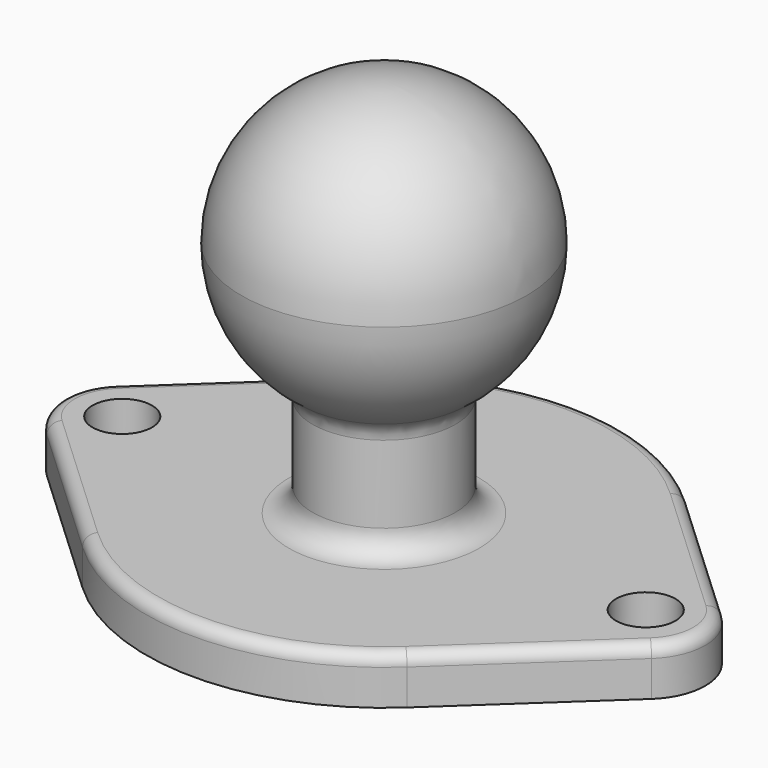
from build123d import *

# Parameters (mm, degrees)
F0_R     = 3.96875
F1_DEPTH = 6.35
F4_DEPTH = 15.2522160579
F5_R     = 1.6002
F6_R     = 3.175


with BuildPart() as f1:
    # F0 (on Top) → F1 (new body)
    with BuildSketch(Plane.XY):
        with BuildLine():
            Line((40.3369318182, 5.8064533276), (21.6477272727, 23.2258133103))
            ThreePointArc((21.6477272727, 23.2258133103), (11.6327754082, 29.5421907837), (0, 31.75))
            ThreePointArc((0, 31.75), (-11.6327754082, 29.5421907837), (-21.6477272727, 23.2258133103))
            Line((-21.6477272727, 23.2258133103), (-40.3369318182, 5.8064533276))
            ThreePointArc((-40.3369318182, 5.8064533276), (-42.8625, 0), (-40.3369318182, -5.8064533276))
            Line((-40.3369318182, -5.8064533276), (-21.6477272727, -23.2258133103))
            ThreePointArc((-21.6477272727, -23.2258133103), (0, -31.75), (21.6477272727, -23.2258133103))
            Line((21.6477272727, -23.2258133103), (40.3369318182, -5.8064533276))
            ThreePointArc((40.3369318182, -5.8064533276), (42.8625, 0), (40.3369318182, 5.8064533276))
        make_face()
        with Locations((-34.925, 0)):
            Circle(F0_R, mode=Mode.SUBTRACT)
        with BuildLine():
            ThreePointArc((9.525, 0), (-6.7351920908, -6.7351920908), (0, 9.525))
            ThreePointArc((0, 9.525), (6.7351920908, 6.7351920908), (9.525, 0))
        make_face(mode=Mode.SUBTRACT)
        with BuildLine():
            ThreePointArc((38.89375, 0), (34.925, -3.96875), (30.95625, 0))
            ThreePointArc((30.95625, 0), (34.925, 3.96875), (38.89375, 0))
        make_face(mode=Mode.SUBTRACT)
        with BuildLine():
            Line((0, 0), (0, 9.525))
            ThreePointArc((0, 9.525), (-6.7351920908, -6.7351920908), (9.525, 0))
            Line((9.525, 0), (0, 0))
        make_face()
        with BuildLine():
            ThreePointArc((9.525, 0), (6.7351920908, 6.7351920908), (0, 9.525))
            Line((0, 9.525), (0, 0))
            Line((0, 0), (9.525, 0))
        make_face()
    extrude(amount=-F1_DEPTH)



with BuildPart() as f3:
    # F2 (on Front) → F3 (revolve)
    with BuildSketch(Plane.XZ):
        with BuildLine():
            Line((0, 50.8), (0, 12.7))
            ThreePointArc((0, 12.7), (13.4703841816, 18.2796158184), (19.05, 31.75))
            ThreePointArc((19.05, 31.75), (13.4703841816, 45.2203841816), (0, 50.8))
        make_face()
    revolve(axis=Axis((0, 0, 25.4), (0, 0, 1)))


with BuildPart() as f1_1:
    add(f1.part)

    add(f3.part)  # F4 merges F3
    # F0 (on Top) → F4 (join, through all)
    with BuildSketch(Plane.XY):
        with BuildLine():
            Line((0, 0), (0, 9.525))
            ThreePointArc((0, 9.525), (-6.7351920908, -6.7351920908), (9.525, 0))
            Line((9.525, 0), (0, 0))
        make_face()
        with BuildLine():
            ThreePointArc((9.525, 0), (6.7351920908, 6.7351920908), (0, 9.525))
            Line((0, 9.525), (0, 0))
            Line((0, 0), (9.525, 0))
        make_face()
    extrude(amount=F4_DEPTH)

    # F5
    f5_edges = [f1_1.edges().sort_by_distance(p)[0] for p in [
        (0, -31.75, 0),
        (42.8625, 0, 0),
        (30.99233, -14.516133, 0),
        (30.99233, 14.516133, 0),
        (0, 31.75, 0),
        (-30.99233, -14.516133, 0),
        (-30.99233, 14.516133, 0),
        (-42.8625, 0, 0),
    ]]
    fillet(f5_edges, radius=F5_R)

    # F6
    f6_edges = [f1_1.edges().sort_by_distance(p)[0] for p in [
        (-9.525, 0, 15.252216),
        (-9.525, 0, 0),
    ]]
    fillet(f6_edges, radius=F6_R)


solid = f1_1.part
